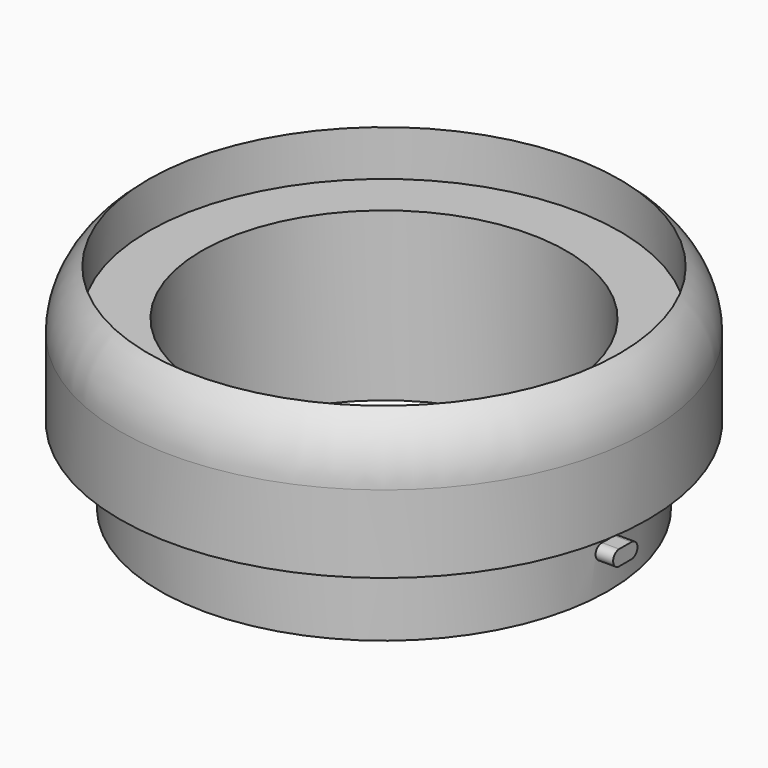
from build123d import *

# Parameters (mm, degrees)
F0_R     = 14.75
F1_DEPTH = 5
F2_R     = 17.375
F3_DEPTH = 9
F5_DEPTH = 15.875
F6_R     = 12
F7_DEPTH = 15
F8_R     = 15.5
F9_DEPTH = 3


# Not quite as in the source:
# - a fillet or chamfer that OpenCascade refuses, or shapes differently, is made with other operations: its cross-section is extruded or revolved along the edge and cut away or added


with BuildPart() as f1:
    # F0 (on Top) → F1 (new body)
    with BuildSketch(Plane.XY):
        Circle(F0_R)
    extrude(amount=F1_DEPTH)

    # F2 (on face) → F3 (join)
    with BuildSketch(Plane.XY.offset(5)):
        Circle(F2_R)
    extrude(amount=F3_DEPTH)

    # F4 (on Right) → F5 (join, symmetric)
    with BuildSketch(Plane.YZ):
        with BuildLine():
            Line((0.5, 3), (-0.5, 3))
            ThreePointArc((-0.5, 3), (-1, 2.5), (-0.5, 2))
            Line((-0.5, 2), (0.5, 2))
            ThreePointArc((0.5, 2), (1, 2.5), (0.5, 3))
        make_face()
    extrude(amount=F5_DEPTH, both=True)

    # F6 (on face) → F7 (cut)
    with BuildSketch(Plane(origin=(0, 0, 0), x_dir=(1, 0, 0), z_dir=(0, 0, -1))):
        Circle(F6_R)
    extrude(amount=-F7_DEPTH, mode=Mode.SUBTRACT)

    # F8 (on face) → F9 (cut)
    with BuildSketch(Plane.XY.offset(14)):
        Circle(F8_R)
    extrude(amount=-F9_DEPTH, mode=Mode.SUBTRACT)

    # F10: fillet of radius 5 on 1 edges, made by hand

    # F10_s1 → F10_t2 (revolve, cut)
    with BuildSketch(Plane.XZ):
        with BuildLine():
            ThreePointArc((17.375, 10.096876251), (16.8819390943, 12.2619397605), (15.5, 14))
            Line((15.5, 14), (17.375, 14))
            Line((17.375, 14), (17.375, 10.096876251))
        make_face()
    revolve(axis=Axis((0, 0, 14), (0, 0, 1)), mode=Mode.SUBTRACT)


solid = f1.part
